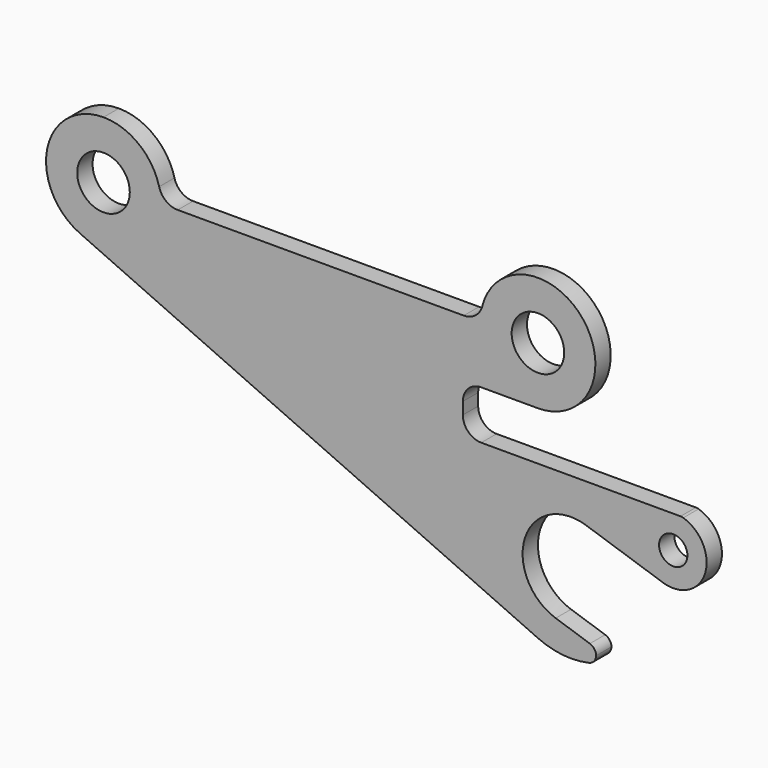
from build123d import *

# Parameters (mm, degrees)
F0_R        = 2.3495
F0_R_2      = 4.3561
F1_DEPTH    = 3.175
F2_T1_DEPTH = 8.6796915338
F2_T3_DEPTH = 9.317688033
F3_R        = 3.048
F4_R        = 3.175
F5_R        = 1.524


# Not quite as in the source:
# - a fillet or chamfer that OpenCascade refuses, or shapes differently, is made with other operations: its cross-section is extruded or revolved along the edge and cut away or added


with BuildPart() as f1:
    # F0 (on Front) → F1 (new body)
    with BuildSketch(Plane.XZ):
        with BuildLine():
            Line((-17.907, 13.9954), (-17.907, 22.0726))
            Line((-17.907, 22.0726), (-5.461, 22.0726))
            ThreePointArc((-5.461, 22.0726), (4.064, 31.5976), (-5.461, 41.1226))
            ThreePointArc((-5.461, 41.1226), (-12.1961920908, 38.3327920908), (-14.986, 31.5976))
            Line((-14.986, 31.5976), (-67.945, 31.5976))
            ThreePointArc((-67.945, 31.5976), (-70.7348079092, 38.3327920908), (-77.47, 41.1226))
            ThreePointArc((-77.47, 41.1226), (-86.7805213206, 33.6075297847), (-81.3993425959, 22.9208556933))
            Line((-81.3993425959, 22.9208556933), (-5.461, -11.4685135998))
            ThreePointArc((-5.461, -11.4685135998), (-0.6838491315, -12.6351736228), (4.191, -11.9885578365))
            Line((4.191, -11.9885578365), (4.191, -9.8147056722))
            Line((4.191, -9.8147056722), (-2.5137480378, -7.5958588588))
            ThreePointArc((-2.5137480378, -7.5958588588), (-7.5958588588, 2.5137480378), (2.5137480378, 7.5958588588))
            Line((2.5137480378, 7.5958588588), (15.2275267548, 3.3884035996))
            ThreePointArc((15.2275267548, 3.3884035996), (22.2730028192, 7.0612251677), (18.3941407903, 13.9954))
            Line((18.3941407903, 13.9954), (-17.907, 13.9954))
        make_face()
        with Locations((16.9672, 8.6452202067)):
            Circle(F0_R, mode=Mode.SUBTRACT)
        with Locations((-77.47, 31.5976)):
            Circle(F0_R_2, mode=Mode.SUBTRACT)
        with Locations((-5.461, 31.5976)):
            Circle(F0_R_2, mode=Mode.SUBTRACT)
    extrude(amount=F1_DEPTH)

    # F2: fillet of radius 1.524 on 2 edges, made by hand

    # F2_s2 → F2_t1 (cut)
    with BuildSketch(Plane.XZ.offset(-2.7523457669)):
        with BuildLine():
            ThreePointArc((3.1458091501, -9.4688137202), (3.9023706215, -10.0232116691), (4.191, -10.915643979))
            Line((4.191, -10.915643979), (4.191, -9.8147056722))
            Line((4.191, -9.8147056722), (3.1458091501, -9.4688137202))
        make_face()
    extrude(amount=F2_T1_DEPTH, mode=Mode.SUBTRACT)

    # F2_s4 → F2_t3 (cut)
    with BuildSketch(Plane.XZ.offset(-3.0713440165)):
        with BuildLine():
            ThreePointArc((4.191, -10.8324529742), (3.8589330034, -11.7821222406), (3.0074413182, -12.3179413481))
            ThreePointArc((3.0074413182, -12.3179413481), (3.6030210464, -12.1669053498), (4.191, -11.9885578365))
            Line((4.191, -11.9885578365), (4.191, -10.8324529742))
        make_face()
    extrude(amount=F2_T3_DEPTH, mode=Mode.SUBTRACT)

    # F3
    f3_edges = [f1.edges().sort_by_distance(p)[0] for p in [
        (-17.907, -1.5875, 22.0726),
        (-17.907, -1.5875, 13.9954),
    ]]
    fillet(f3_edges, radius=F3_R)

    # F4
    f4_edges = [f1.edges().sort_by_distance(p)[0] for p in [
        (-67.945, -1.5875, 31.5976),
        (-14.986, -1.5875, 31.5976),
    ]]
    fillet(f4_edges, radius=F4_R)

    # F5
    f5_edges = [f1.edges().sort_by_distance(p)[0] for p in [
        (18.394141, -1.5875, 13.9954),
    ]]
    fillet(f5_edges, radius=F5_R)


solid = f1.part
